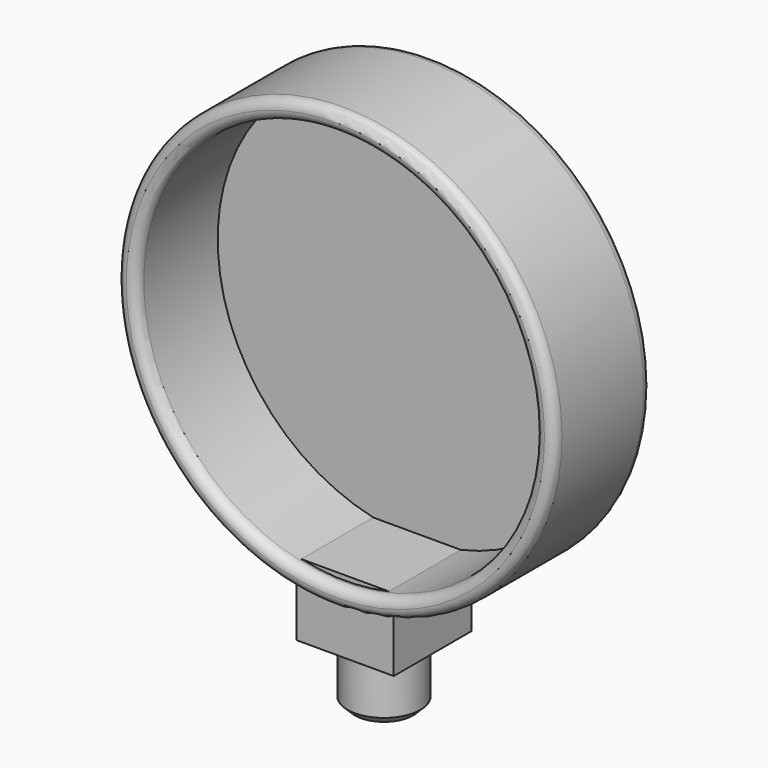
from build123d import *

# Parameters (mm, degrees)
F0_R     = 57.15
F1_DEPTH = 31.75
F2_T     = -5.08
F4_W     = 25.4
F4_H     = 25.4
F5_DEPTH = 19.05
F6_R     = 2.53999
F7_R     = 9.525
F8_DEPTH = 15.875
F9_SIZE  = 1.905


# Not quite as in the source:
# - a fillet or chamfer is up to 0.001 mm smaller than in the source, because OpenCascade refuses the exact size


with BuildPart() as f1:
    # F0 (on Front) → F1 (new body)
    with BuildSketch(Plane.XZ):
        Circle(F0_R)
    extrude(amount=F1_DEPTH)

    # F2
    f2_openings = [f1.faces().sort_by_distance(p)[0] for p in [
        (0, -31.75, 0),
    ]]
    offset(amount=F2_T, openings=f2_openings)

    # F4 (on offset) → F5 (join)
    with BuildSketch(Plane.XY.offset(-50.8)):
        with Locations((0, -15.875)):
            Rectangle(F4_W, F4_H)
    extrude(amount=-F5_DEPTH)

    # F6 (radius 2.54 in the source; OpenCascade refuses exactly that, so slightly less here)
    f6_edges = [f1.edges().sort_by_distance(p)[0] for p in [
        (-57.15, -31.75, 0),
        (-52.07, -31.75, 0),
        (-57.15, 0, 0),
    ]]
    fillet(f6_edges, radius=F6_R)

    # F7 (on face) → F8 (join)
    with BuildSketch(Plane(origin=(0, 0, -69.85), x_dir=(1, 0, 0), z_dir=(0, 0, -1))):
        with Locations((0, 15.875)):
            Circle(F7_R)
    extrude(amount=F8_DEPTH)

    # F9
    f9_edges = [f1.edges().sort_by_distance(p)[0] for p in [
        (-9.525, -15.875, -85.725),
    ]]
    chamfer(f9_edges, length=F9_SIZE)


solid = f1.part
